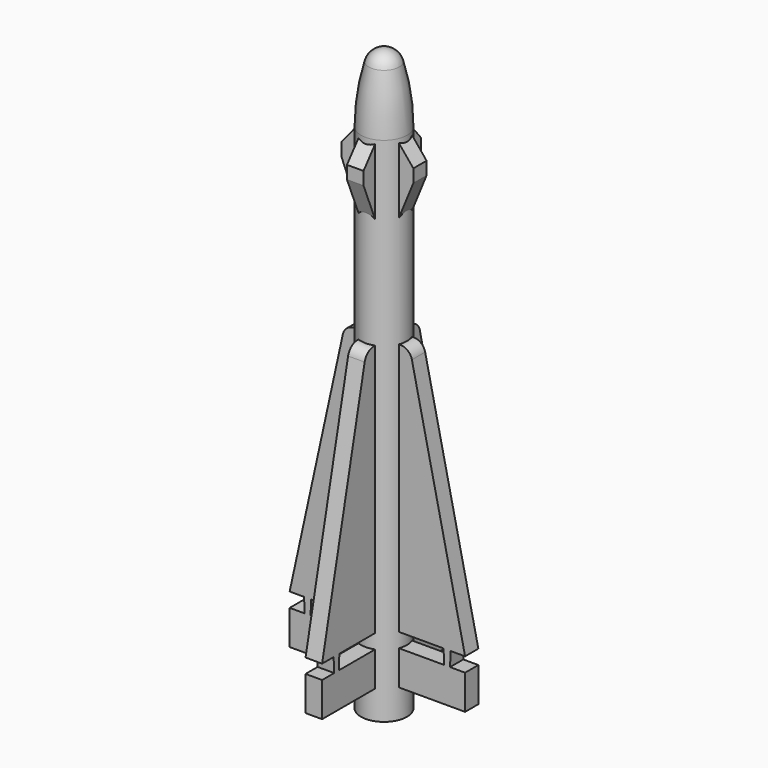
from build123d import *

# Parameters (mm, degrees)
F3_DEPTH = 0.2
F4_COUNT = 4


# Not quite as in the source:
# - a feature names something its author has since deleted; it is built from what else it names


with BuildPart() as f1:
    # F0 (on Front) → F1 (revolve)
    with BuildSketch(Plane.XZ):
        with BuildLine():
            Line((0, 14.0277777778), (0, 0))
            Line((0, 0), (0.5555555556, 0))
            Line((0.5555555556, 0), (0.5555555556, 12.3611111111))
            ThreePointArc((0.5555555556, 12.3611111111), (0.5078793667, 13.0620116793), (0.3657291084, 13.75))
            ThreePointArc((0.3657291084, 13.75), (0.2296291982, 13.9504603784), (0, 14.0277777778))
        make_face()
    revolve(axis=Axis((0, 0, 7.0138888889), (0, 0, 1)))

    # F2 (on Front) → F3 (join, symmetric)
    with BuildSketch(Plane.XZ):
        with BuildLine():
            Line((0, 12.6567901235), (0, 0.6944444444))
            Line((0, 0.6944444444), (2.1180555556, 0.6944444444))
            Line((2.1180555556, 0.6944444444), (2.1180555556, 1.5277777778))
            Line((2.1180555556, 1.5277777778), (1.7534722222, 1.5277777778))
            Line((1.7534722222, 1.5277777778), (1.6145833333, 1.5277777778))
            Line((1.6145833333, 1.5277777778), (0.4, 1.5277777778))
            Line((0.4, 1.5277777778), (0.4, 1.875))
            Line((0.4, 1.875), (1.5972222222, 1.875))
            Line((1.5972222222, 1.875), (1.7708333333, 1.875))
            Line((1.7708333333, 1.875), (2.1180555556, 1.875))
            Line((2.1180555556, 1.875), (0.8333333333, 7.7624119633))
            ThreePointArc((0.8333333333, 7.7624119633), (0.7338823641, 7.9232334612), (0.5555555556, 7.9861111111))
            Line((0.5555555556, 7.9861111111), (0.2, 7.9861111111))
            Line((0.2, 7.9861111111), (0.2, 9.8947530864))
            Line((0.2, 9.8947530864), (0.8680555556, 11.5277777778))
            Line((0.8680555556, 11.5277777778), (0.8680555556, 11.8402777778))
            Line((0.8680555556, 11.8402777778), (0.2, 12.6567901235))
            Line((0.2, 12.6567901235), (0, 12.6567901235))
        make_face()
        Polygon((1.6145833333, 1.5277777778), (1.7534722222, 1.5277777778), (1.7708333333, 1.875), (1.5972222222, 1.875), align=None)
    extrude(amount=F3_DEPTH, both=True)

    # F4: F1 ×4 about axis
    f4_axis = Axis((0, 0, 0), (0, 0, 1))


with BuildPart() as f1_1:
    add(f1.part)
    for i in range(1, F4_COUNT):
        add(f1.part.rotate(f4_axis, i * 360 / F4_COUNT))


solid = f1_1.part
